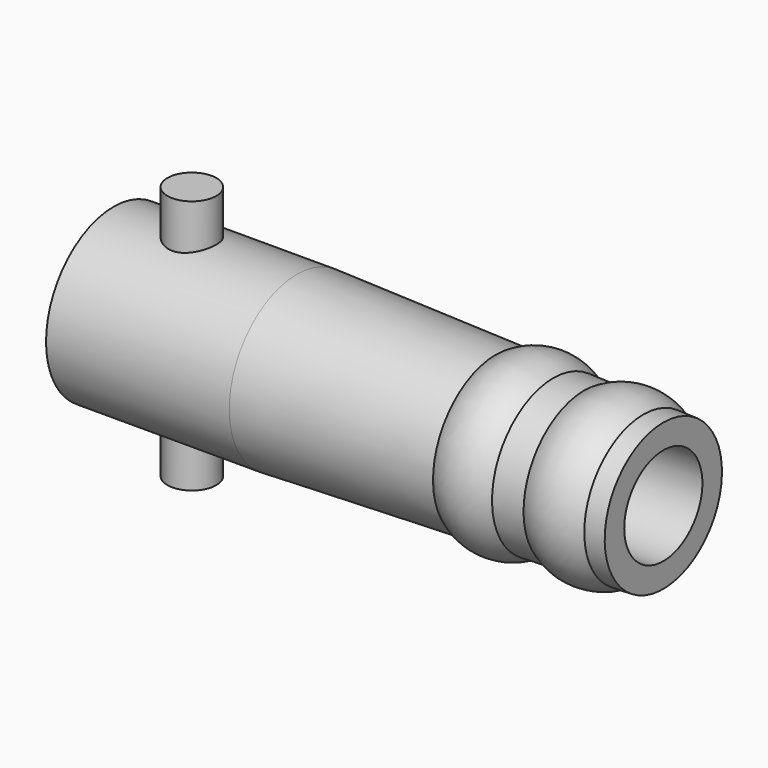
from build123d import *

# Parameters (mm, degrees)
F4_R     = 4
F5_DEPTH = 45


# Not quite as in the source:
# - a feature names something its author has since deleted; it is built from what else it names


with BuildPart() as f1:
    # F0 (on Front) → F1 (revolve)
    with BuildSketch(Plane.XZ):
        with BuildLine():
            ThreePointArc((1.311079303, 6.2763909436), (-1.0236192616, 7.0769066725), (-3.4030299061, 6.4211263706))
            Line((-3.4030299061, 6.4211263706), (1.311079303, 6.2763909436))
        make_face()
        with BuildLine():
            Line((3.831038924, 6.1990216219), (8.6828378167, 6.0500587631))
            ThreePointArc((8.6828378167, 6.0500587631), (6.2786539333, 6.8318275323), (3.831038924, 6.1990216219))
        make_face()
        Polygon((-34.6867218614, 6.921078112), (-34.6867218614, 0), (10.3132781386, 0), (10.3132781386, 6), (8.6828378167, 6.0500587631), (3.831038924, 6.1990216219), (1.311079303, 6.2763909436), (-3.4030299061, 6.4211263706), (-19.6867218614, 6.921078112), align=None)
    revolve(axis=Axis((-12.1867218614, 0, 0), (1, 0, 0)))

    # F2 (on Front) → F3 (revolve)
    with BuildSketch(Plane.XZ):
        Polygon((-30.2853044122, -6.0204798356), (-30.2853044122, -6.921078112), (-30.2853044122, -10.421078112), (-28.2853044122, -10.421078112), (-28.2853044122, -6.921078112), (-28.2853044122, -6.0204798356), align=None)
        Polygon((-28.2853044122, 6.921078112), (-28.2853044122, 10.421078112), (-30.2853044122, 10.421078112), (-30.2853044122, 6.921078112), (-30.2853044122, 5.468968302), (-28.2853044122, 5.468968302), align=None)
    revolve(axis=Axis((-28.2853044122, 0, 8.671078112), (0, 0, -1)))

    # F4 (on face) → F5 (cut, through all)
    with BuildSketch(Plane(origin=(-34.6867218614, 0, 0), x_dir=(0, -1, 0), z_dir=(-1, 0, 0))):
        Circle(F4_R)
    extrude(amount=-F5_DEPTH, mode=Mode.SUBTRACT)


solid = f1.part
